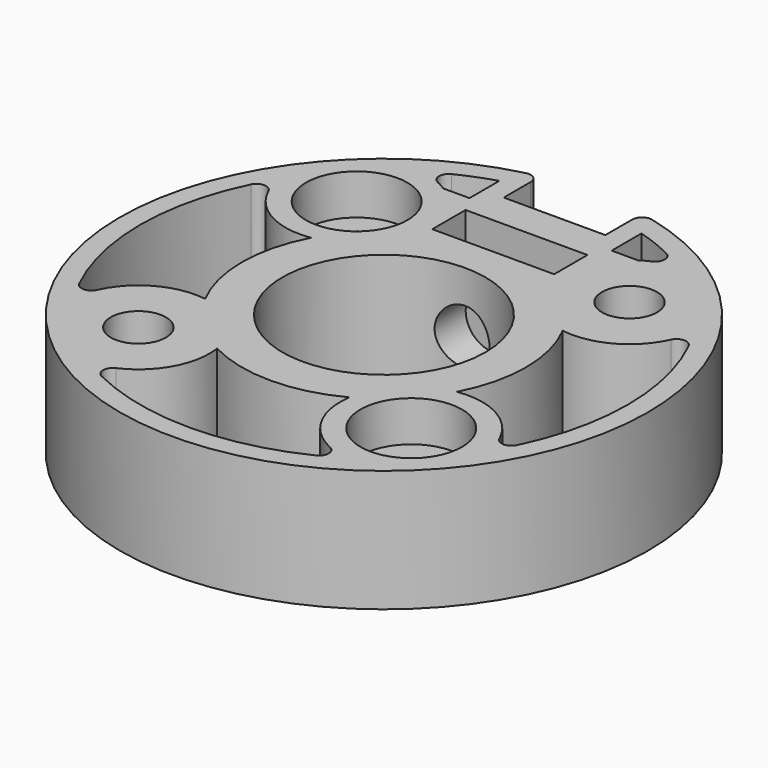
from build123d import *

# Parameters (mm, degrees)
F0_R            = 2.15265
F0_R_2          = 7.9375
F1_DEPTH        = 9.525
F2_R            = 2.15265
F3_REACH        = 43.3958636501
F5_R            = 3.96875
F6_DEPTH        = 3.175
F8_DEPTH        = 9.525
F8_COPIES_COUNT = 3
F8_COPIES_ANGLE = 180
F9_R            = 2.15265
F10_REACH       = 43.3958636501
F12_DEPTH       = 9.525
F13_R           = 0.762


# Not quite as in the source:
# - a pattern or mirror of a feature is missing from the dataset's text; its kind, count and spacing are read off the source's solid


with BuildPart() as f1:
    # F0 (on Top) → F1 (new body)
    with BuildSketch(Plane.XY):
        with BuildLine():
            Line((3.96875, 16.66875), (0, 16.66875))
            Line((0, 16.66875), (-3.96875, 16.66875))
            Line((-3.96875, 16.66875), (-3.96875, 20.2522944302))
            ThreePointArc((-3.96875, 20.2522944302), (0, -20.6375), (3.96875, 20.2522944302))
            Line((3.96875, 20.2522944302), (3.96875, 16.66875))
        make_face()
        with Locations((-10.6640541438, -10.6640541438)):
            Circle(F0_R, mode=Mode.SUBTRACT)
        with Locations((10.6640541438, -10.6640541438)):
            Circle(F0_R, mode=Mode.SUBTRACT)
        with Locations((-10.6640541438, 10.6640541438)):
            Circle(F0_R, mode=Mode.SUBTRACT)
        Circle(F0_R_2, mode=Mode.SUBTRACT)
        Polygon((-4.7625, 13.928725), (0, 13.928725), (4.7625, 13.928725), (4.7625, 10.677525), (-4.7625, 10.677525), align=None, mode=Mode.SUBTRACT)
        with Locations((10.6640541438, 10.6640541438)):
            Circle(F0_R, mode=Mode.SUBTRACT)
    extrude(amount=F1_DEPTH)

    f3_end = f1.faces().sort_by_distance((-7.9375, 0, 4.7625))[0]
    # F2 (on face) → F3 (cut, up to a face of the model that its end follows)
    with BuildSketch(Plane(origin=(0, 16.66875, 0), x_dir=(-1, 0, 0), z_dir=(0, 1, 0))):
        with Locations((0, 4.7625)):
            Circle(F2_R)
    f3_long = extrude(amount=-F3_REACH, mode=Mode.PRIVATE)
    add(split(f3_long, bisect_by=f3_end, keep=Keep.ALL, mode=Mode.PRIVATE).solids().sort_by_distance((0, 16.66875, 4.7625))[0], mode=Mode.SUBTRACT)

    # F5 (on face) → F6 (cut, through all)
    with BuildSketch(Plane.XY.offset(9.525)):
        with Locations((-10.6640541438, 10.6640541438)):
            Circle(F5_R)
        with Locations((10.6640541438, -10.6640541438)):
            Circle(F5_R)
    extrude(amount=-F6_DEPTH, mode=Mode.SUBTRACT)

    # F7 (on face) → F8 (cut, through all)
    with BuildSketch(Plane.XY.offset(9.525)):
        with BuildLine():
            ThreePointArc((-9.836738319, 5.1697423044), (-14.0484138573, 6.2574655095), (-16.1858200979, 10.0459806768))
            ThreePointArc((-16.1858200979, 10.0459806768), (-19.05, 0), (-16.1858200979, -10.0459806768))
            ThreePointArc((-16.1858200979, -10.0459806768), (-14.0484138573, -6.2574655095), (-9.836738319, -5.1697423044))
            ThreePointArc((-9.836738319, -5.1697423044), (-11.1125, 0), (-9.836738319, 5.1697423044))
        make_face()
    f8 = extrude(amount=-F8_DEPTH, mode=Mode.SUBTRACT)

    # F8_copies: F8 ×3 about axis
    f8_copies_axis = Axis((0, 0, 0), (0, 0, 1))
    for i in range(1, F8_COPIES_COUNT):
        add(f8.rotate(f8_copies_axis, i * F8_COPIES_ANGLE / (F8_COPIES_COUNT - 1)), mode=Mode.SUBTRACT)

    f10_end = f1.faces().sort_by_distance((-7.9375, 0, 4.7625))[0]
    # F9 (on face) → F10 (cut, up to a face of the model that its end follows)
    with BuildSketch(Plane(origin=(0, 16.66875, 0), x_dir=(-1, 0, 0), z_dir=(0, 1, 0))):
        with Locations((0, 4.7625)):
            Circle(F9_R)
    f10_long = extrude(amount=-F10_REACH, mode=Mode.PRIVATE)
    add(split(f10_long, bisect_by=f10_end, keep=Keep.TOP, mode=Mode.PRIVATE), mode=Mode.SUBTRACT)

    # F11 (on face) → F12 (cut, through all)
    with BuildSketch(Plane.XY.offset(9.525)):
        with BuildLine():
            ThreePointArc((-10.0459806768, 16.1858200979), (-8.7741608818, 15.8890151504), (-7.6067543541, 15.3035403285))
            Line((-7.6067543541, 15.3035403285), (-5.55625, 15.3035403285))
            Line((-5.55625, 15.3035403285), (-5.55625, 18.2217064497))
            ThreePointArc((-5.55625, 18.2217064497), (-7.8672491274, 17.3496078102), (-10.0459806768, 16.1858200979))
        make_face()
        with BuildLine():
            ThreePointArc((10.0459806768, 16.1858200979), (7.8672491274, 17.3496078102), (5.55625, 18.2217064497))
            Line((5.55625, 18.2217064497), (5.55625, 15.3035403285))
            Line((5.55625, 15.3035403285), (7.6067543541, 15.3035403285))
            ThreePointArc((7.6067543541, 15.3035403285), (8.7741608818, 15.8890151504), (10.0459806768, 16.1858200979))
        make_face()
    extrude(amount=-F12_DEPTH, mode=Mode.SUBTRACT)

    # F13
    f13_edges = [f1.edges().sort_by_distance(p)[0] for p in [
        (-16.18582, -10.045981, 4.7625),
        (-16.18582, 10.045981, 4.7625),
        (10.045981, 16.18582, 4.7625),
        (3.96875, 20.252294, 4.7625),
        (-3.96875, 20.252294, 4.7625),
        (-10.045981, 16.18582, 4.7625),
        (10.045981, -16.18582, 4.7625),
        (-10.045981, -16.18582, 4.7625),
        (16.18582, 10.045981, 4.7625),
        (16.18582, -10.045981, 4.7625),
    ]]
    fillet(f13_edges, radius=F13_R)


solid = f1.part
